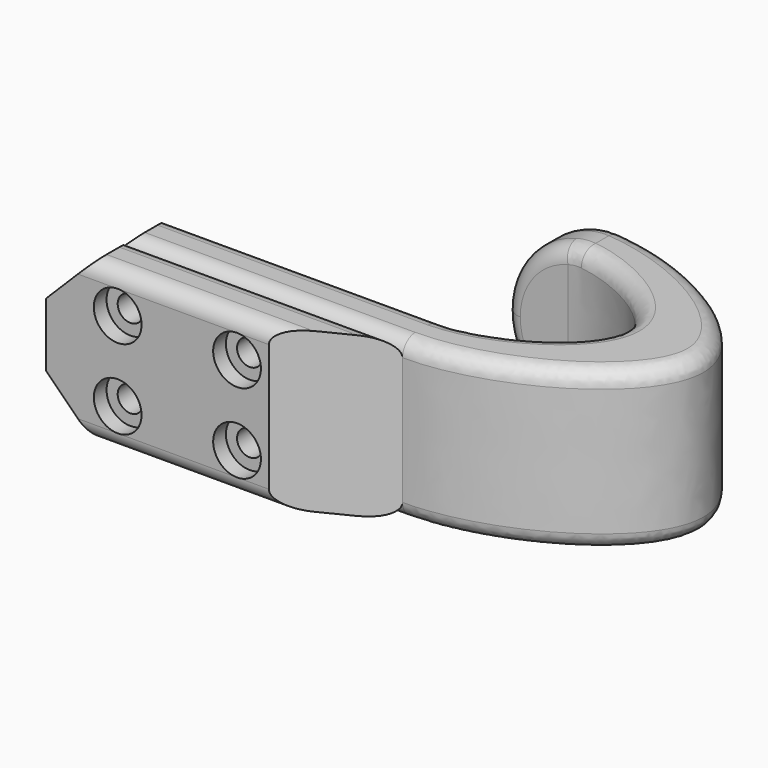
from build123d import *

# Parameters (mm, degrees)
F1_DEPTH        = 20
F2_R            = 9.99999
F3_R            = 2
F5_DEPTH        = 40
F6_DEPTH        = 35
F7_R            = 2
F8_T1_DEPTH     = 78.1558929709
F9_T1_DEPTH     = 32.8601958556
F9_2_T1_DEPTH   = 32.8601958556
F11_D           = 3.2
F11_DEPTH       = 6
F11_CBORE_D     = 6
F11_CBORE_DEPTH = 2
F11_TIP         = 0.9613769904
F12_D           = 2
F12_DEPTH       = 25
F12_TIP         = 0.600860619


# Not quite as in the source:
# - a fillet or chamfer that OpenCascade refuses, or shapes differently, is made with other operations: its cross-section is extruded or revolved along the edge and cut away or added
# - a fillet or chamfer is up to 0.001 mm smaller than in the source, because OpenCascade refuses the exact size


with BuildPart() as f1:
    # F0 (on Top) → F1 (new body)
    with BuildSketch(Plane.XY):
        with BuildLine():
            Line((0, 6), (0, 0))
            Line((0, 0), (40, 0))
            add(Edge.make_bspline(
                [(40, 32.0000038027), (51, 32.0000038027), (79, 15.9999527813), (51, 0), (40, 0)],
                knots=[0, 0, 0, 0, 0.5000001305, 1, 1, 1, 1], degree=3))
            Line((40, 32.0000038027), (32, 32.0000038027))
            Line((32, 32.0000038027), (32, 26.0000038027))
            Line((32, 26.0000038027), (40, 26.0000038027))
            add(Edge.make_bspline(
                [(40, 26.0000038027), (46, 26.0000038027), (64, 15.999953273), (46, 6), (40, 6)],
                knots=[0, 0, 0, 0, 0.500000221, 1, 1, 1, 1], degree=3))
            Line((40, 6), (0, 6))
        make_face()
    extrude(amount=F1_DEPTH)

    # F2 (radius 10 in the source; OpenCascade refuses exactly that, so slightly less here)
    f2_edges = [f1.edges().sort_by_distance(p)[0] for p in [
        (32, 29.000004, 0),
        (32, 29.000004, 20),
    ]]
    fillet(f2_edges, radius=F2_R)

    # F3
    f3_edges = [f1.edges().sort_by_distance(p)[0] for p in [
        (20, 6, 0),
        (20, 0, 20),
    ]]
    fillet(f3_edges, radius=F3_R)


with BuildPart() as f5:
    # F4 (on face) → F5 (new body)
    with BuildSketch(Plane(origin=(0, 0, 0), x_dir=(0, -1, 0), z_dir=(-1, 0, 0))):
        with BuildLine():
            ThreePointArc((0, 11.9), (1.3435028843, 11.3435028843), (1.9, 10))
            ThreePointArc((1.9, 10), (1.3435028843, 8.6564971157), (0, 8.1))
            Line((0, 8.1), (0, 2))
            Line((0, 2), (0, 0))
            Line((0, 0), (6, 0))
            Line((6, 0), (6, 20))
            Line((6, 20), (0, 20))
            Line((0, 20), (0, 18))
            Line((0, 18), (0, 11.9))
        make_face()
        with BuildLine():
            ThreePointArc((0, 8.1), (1.3435028843, 8.6564971157), (1.9, 10))
            ThreePointArc((1.9, 10), (1.3435028843, 11.3435028843), (0, 11.9))
            Line((0, 11.9), (0, 8.1))
        make_face()
    extrude(amount=-F5_DEPTH)


with BuildPart() as f6_tool:
    # F4 (on face) → F6 (new body)
    with BuildSketch(Plane(origin=(0, 0, 0), x_dir=(0, -1, 0), z_dir=(-1, 0, 0))):
        with BuildLine():
            Line((0, 8.1), (0, 11.9))
            ThreePointArc((0, 11.9), (-1.9, 10), (0, 8.1))
        make_face()
        with BuildLine():
            ThreePointArc((0, 8.1), (1.3435028843, 8.6564971157), (1.9, 10))
            ThreePointArc((1.9, 10), (1.3435028843, 11.3435028843), (0, 11.9))
            Line((0, 11.9), (0, 8.1))
        make_face()
    extrude(amount=-F6_DEPTH)


with BuildPart() as f1_1:
    add(f1.part)

    # F6: cut by f6_tool
    add(f6_tool.part, mode=Mode.SUBTRACT)

    # F9: chamfer of 6 on 2 edges, made by hand

    # F9_s2 → F9_t1 (cut)
    with BuildSketch(Plane.XZ.offset(-19.4300979278)):
        Polygon((6, 0), (0, 6), (0, 0), align=None)
        Polygon((6, 20), (0, 14), (0, 20), align=None)
    extrude(amount=F9_T1_DEPTH, mode=Mode.SUBTRACT)

    # F12
    with Locations(Plane.XZ.offset(6)):
        with Locations((24, 15), (24, 5), (9, 5), (9, 15)):
            Hole(F12_D / 2, depth=F12_DEPTH)
            with Locations((0, 0, -(F12_DEPTH + F12_TIP / 2))):  # 118° drill point
                Cone(0, F12_D / 2, F12_TIP, mode=Mode.SUBTRACT)


with BuildPart() as f5_1:
    add(f5.part)

    # F6: cut by f6_tool
    add(f6_tool.part, mode=Mode.SUBTRACT)

    # F7
    f7_edges = [f5_1.edges().sort_by_distance(p)[0] for p in [
        (20, 0, 0),
        (20, -6, 0),
        (20, 0, 20),
        (20, -6, 20),
    ]]
    fillet(f7_edges, radius=F7_R)

    # F8: chamfer of 12 x 6 on 1 edges, made by hand

    # F8_s2 → F8_t1 (cut)
    with BuildSketch(Plane.XY.offset(-29.0779464854)):
        Polygon((40, 0), (28, -6), (40, -6), align=None)
    extrude(amount=F8_T1_DEPTH, mode=Mode.SUBTRACT)

    # F9#2: chamfer of 6 on 2 edges, made by hand

    # F9_2_s2 → F9_2_t1 (cut)
    with BuildSketch(Plane.XZ.offset(-13.4300979278)):
        Polygon((6, 0), (0, 6), (0, 0), align=None)
        Polygon((0, 14), (6, 20), (0, 20), align=None)
    extrude(amount=F9_2_T1_DEPTH, mode=Mode.SUBTRACT)

    # F11
    with Locations(Plane.XZ.offset(6)):
        with Locations((24, 15), (24, 5), (9, 5), (9, 15)):
            CounterBoreHole(F11_D / 2, F11_CBORE_D / 2, F11_CBORE_DEPTH, depth=F11_DEPTH)
            with Locations((0, 0, -(F11_DEPTH + F11_TIP / 2))):  # 118° drill point
                Cone(0, F11_D / 2, F11_TIP, mode=Mode.SUBTRACT)


solid = Compound([f1_1.part, f5_1.part])
